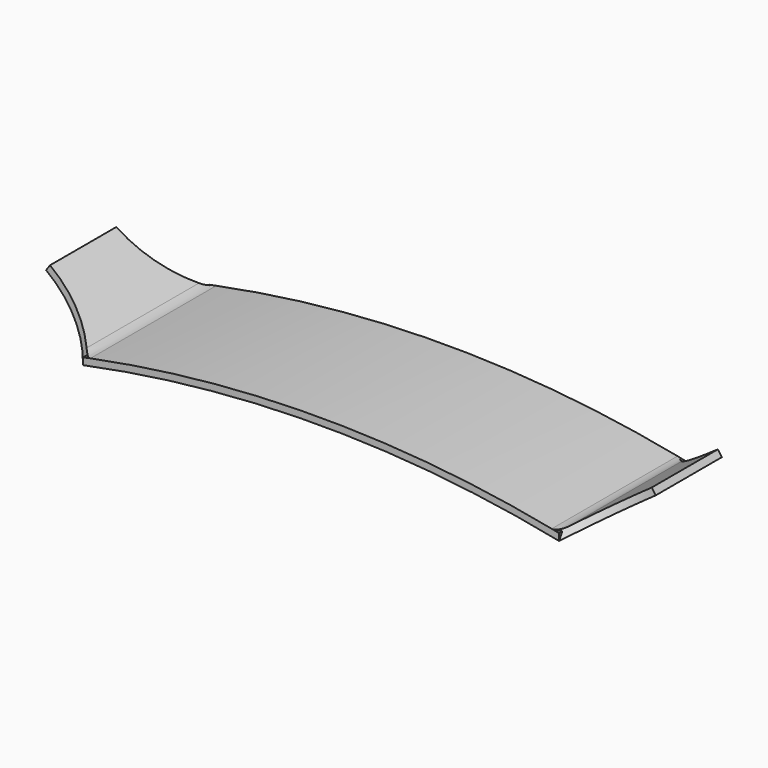
from build123d import *

# Parameters (mm, degrees)
F1_DEPTH      = 114
F3_DEPTH      = 10
F4_ANGLE      = 35
F9_T4_DEPTH   = 262.5652555071
F9_S5_R       = 167.9439583926
F9_T6_DEPTH   = 133
F9_S7_R       = 167.9439583926
F9_T8_DEPTH   = 133
F10_T4_DEPTH  = 262.4928960507
F10_S7_R      = 167.9439583926
F10_T8_DEPTH  = 133
F10_S9_R      = 167.9439583926
F10_T10_DEPTH = 133


# Not quite as in the source:
# - a fillet or chamfer that OpenCascade refuses, or shapes differently, is made with other operations: its cross-section is extruded or revolved along the edge and cut away or added


with BuildPart() as f1:
    # F0 (on Front) → F1 (new body, symmetric)
    with BuildSketch(Plane.XZ):
        with BuildLine():
            ThreePointArc((-332.1381211281, 0), (12.8618788719, 35.0482151539), (357.8618788719, 0))
            Line((357.8618788719, 0), (357.8618788719, 10))
            ThreePointArc((357.8618788719, 10), (12.8618788719, 45.0482151539), (-332.1381211281, 10))
            Line((-332.1381211281, 10), (-332.1381211281, 0))
        make_face()
    extrude(amount=F1_DEPTH, both=True)


with BuildPart() as f3:
    # F2 (on Top) → F3 (new body)
    with BuildSketch(Plane.XY):
        with BuildLine():
            ThreePointArc((123.1073781215, 58.2170858979), (58.6810369853, 73.3595252621), (5.1073781215, 112.2170853764))
            Line((5.1073781215, 112.2170853764), (5.1073781215, -115.7829146236))
            ThreePointArc((5.1073781215, -115.7829146236), (58.6810369853, -76.9253545093), (123.1073781215, -61.7829151452))
            Line((123.1073781215, -61.7829151452), (123.1073781215, 58.2170858979))
        make_face()
    extrude(amount=F3_DEPTH)


with BuildPart() as f3_1:
    # F4: moved
    add(f3.part.rotate(Axis((5.1073781215, -1.7829146236, 0), (0, -1, 0)), F4_ANGLE))


with BuildPart() as f3_2:
    # F5: moved
    add(f3_1.part.moved(Location((352.9, 1.9, 0))))


with BuildPart() as f6_1:
    # F6: instance of F3
    add(f3_2.part.mirror(Plane.YZ))


with BuildPart() as f6_1_1:
    # F7: moved
    add(f6_1.part.moved(Location((25.6, 0, 0))))

    # F8: union F1, F3
    add(f1.part)
    add(f3_2.part)

    # F9: fillet of radius 20 on 1 edges, made by hand


with BuildPart() as f9_tool2:
    # F9_s3 → F9_t4 (new body)
    with BuildSketch(Plane.XZ.offset(-131.39971313)):
        with BuildLine():
            add(Edge.make_bspline(
                [(-336.9253398984, 15.3712567812), (-329.9304765428, 10.4734007308), (-321.5551366342, 12.1379693445)],
                knots=[0, 0, 0, 1, 1, 1], degree=2, weights=[1, 1, 1]))
            ThreePointArc((-321.5551366342, 12.1379693445), (-325.7318557218, 11.3024702142), (-329.9064875028, 10.4566034242))
            Line((-329.9064875028, 10.4566034242), (-336.9253398984, 15.3712567812))
        make_face()
    extrude(amount=F9_T4_DEPTH)

    # F9_s5 → F9_t6 (cut, symmetric)
    with BuildSketch(Plane(origin=(-102.2686786014, 0, -146.0548094967), x_dir=(0, 1, 0), z_dir=(-0.5735764364, 0, -0.8191520443))):
        with Locations((-227.7381227134, -395.7513456072)):
            Circle(F9_S5_R)
    extrude(amount=F9_T6_DEPTH, both=True, mode=Mode.SUBTRACT)

    # F9_s7 → F9_t8 (cut, symmetric)
    with BuildSketch(Plane(origin=(-102.2686786014, 0, -146.0548094967), x_dir=(0, 1, 0), z_dir=(-0.5735764364, 0, -0.8191520443))):
        with Locations((227.9722934661, -395.7513456072)):
            Circle(F9_S7_R)
    extrude(amount=F9_T8_DEPTH, both=True, mode=Mode.SUBTRACT)

    split(bisect_by=Plane.XZ.offset(114), keep=Keep.BOTTOM)

    split(bisect_by=Plane.XZ.offset(-114), keep=Keep.TOP)


with BuildPart() as f6_1_2:
    add(f6_1_1.part)

    # F9_t1: union F9_tool2
    add(f9_tool2.part)

    # F10: fillet of radius 20 on 1 edges, made by hand


with BuildPart() as f10_tool2:
    # F10_s3 → F10_t4 (new body)
    with BuildSketch(Plane.XZ.offset(-131.3635334017)):
        with BuildLine():
            add(Edge.make_bspline(
                [(347.1836055083, 12.1569048592), (355.5583829749, 10.492941025), (362.5526978832, 15.3904130484)],
                knots=[0, 0, 0, 1, 1, 1], degree=2, weights=[1, 1, 1]))
            Line((362.5526978832, 15.3904130484), (355.5343963998, 10.4761454443))
            ThreePointArc((355.5343963998, 10.4761454443), (351.360044149, 11.3217082271), (347.1836055083, 12.1569048592))
        make_face()
    extrude(amount=F10_T4_DEPTH)

    split(bisect_by=Plane.XZ.offset(114), keep=Keep.BOTTOM)

    split(bisect_by=Plane.XZ.offset(-114), keep=Keep.TOP)

    # F10_s7 → F10_t8 (cut, symmetric)
    with BuildSketch(Plane(origin=(110.6428945721, 0, -158.0144293433), x_dir=(0, 1, 0), z_dir=(0.5735764364, 0, -0.8191520443))):
        with Locations((227.9722934661, 416.721637941)):
            Circle(F10_S7_R)
    extrude(amount=F10_T8_DEPTH, both=True, mode=Mode.SUBTRACT)

    # F10_s9 → F10_t10 (cut, symmetric)
    with BuildSketch(Plane(origin=(110.6428945721, 0, -158.0144293433), x_dir=(0, 1, 0), z_dir=(0.5735764364, 0, -0.8191520443))):
        with Locations((-227.7381227134, 416.721637941)):
            Circle(F10_S9_R)
    extrude(amount=F10_T10_DEPTH, both=True, mode=Mode.SUBTRACT)


with BuildPart() as f6_1_3:
    add(f6_1_2.part)

    # F10_t1: union F10_tool2
    add(f10_tool2.part)


solid = f6_1_3.part
